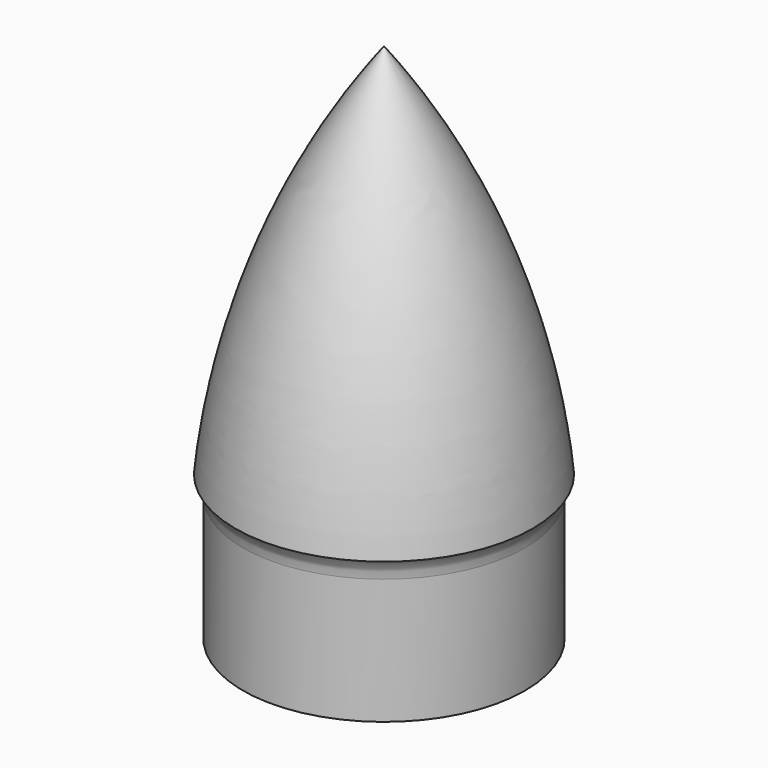
from build123d import *

# Parameters (mm, degrees)
F3_DEPTH = 4


# Not quite as in the source:
# - a fillet or chamfer that OpenCascade refuses, or shapes differently, is made with other operations: its cross-section is extruded or revolved along the edge and cut away or added


with BuildPart() as f1:
    # F0 (on Front) → F1 (revolve)
    with BuildSketch(Plane.XZ):
        with BuildLine():
            Line((0, 3.5), (0, 0))
            Line((0, 0), (24.35, 0))
            Line((24.35, 0), (24.35, 25))
            Line((24.35, 25), (25.62, 25))
            ThreePointArc((25.62, 25), (17.2593424634, 59.2537254448), (0, 90))
            Line((0, 90), (0, 89))
            ThreePointArc((0, 89), (16.3660007492, 59.0312488997), (24.62, 25.8975271136))
            Line((24.62, 25.8975271136), (24.35, 25.8975271136))
            Line((24.35, 25.8975271136), (23.35, 25.8975271136))
            Line((23.35, 25.8975271136), (23.35, 25))
            Line((23.35, 25), (23.35, 3.5))
            Line((23.35, 3.5), (0, 3.5))
        make_face()
    revolve(axis=Axis((0, 0, 45), (0, 0, 1)))

    # F2 (on face) → F3 (cut)
    with BuildSketch(Plane(origin=(0, 0, 0), x_dir=(1, 0, 0), z_dir=(0, 0, -1))):
        Polygon((-5, -10), (-5, 0), (-5, 10), (-12, 10), (-12, -10), align=None)
        Polygon((5, 10), (5, 0), (5, -10), (12, -10), (12, 10), align=None)
    extrude(amount=-F3_DEPTH, mode=Mode.SUBTRACT)

    # F4: fillet of radius 5 on 1 edges, made by hand

    # F4_s1 → F4_t2 (revolve)
    with BuildSketch(Plane.XZ):
        with BuildLine():
            ThreePointArc((24.35, 21.6702702812), (24.6782765493, 23.4521232494), (25.62, 25))
            Line((25.62, 25), (24.35, 25))
            Line((24.35, 25), (24.35, 21.6702702812))
        make_face()
    revolve(axis=Axis((0, 0, 25), (0, 0, 1)))


solid = f1.part
